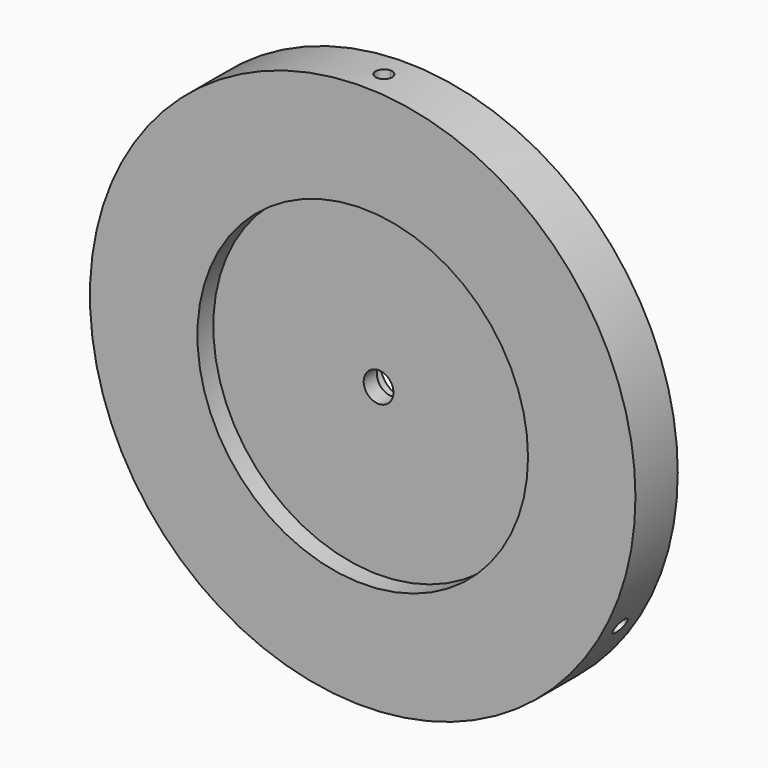
from build123d import *

# Parameters (mm, degrees)
F0_R            = 82.5
F1_DEPTH        = 16
F2_R            = 50
F3_DEPTH        = 6
F6_DEPTH        = 28
F6_COPIES_COUNT = 3
F7_R            = 4.5
F8_DEPTH        = 25
F9_R            = 7.5
F9_R_2          = 4.5
F10_DEPTH       = 5


# Not quite as in the source:
# - a pattern or mirror of a feature is missing from the dataset's text; its kind, count and spacing are read off the source's solid


with BuildPart() as f1:
    # F0 (on Front) → F1 (new body)
    with BuildSketch(Plane.XZ):
        Circle(F0_R)
    extrude(amount=F1_DEPTH)

    # F2 (on face) → F3 (cut)
    with BuildSketch(Plane.XZ.offset(16)):
        Circle(F2_R)
    extrude(amount=-F3_DEPTH, mode=Mode.SUBTRACT)

    # F5 (on offset) → F6 (cut)
    with BuildSketch(Plane.XY.offset(82.5)):
        with BuildLine():
            ThreePointArc((2.5, -8), (1.767766953, -6.232233047), (0, -5.5))
            Line((0, -5.5), (0, -10.5))
            ThreePointArc((0, -10.5), (1.767766953, -9.767766953), (2.5, -8))
        make_face()
        with BuildLine():
            Line((0, -10.5), (0, -5.5))
            ThreePointArc((0, -5.5), (-2.5, -8), (0, -10.5))
        make_face()
    f6 = extrude(amount=-F6_DEPTH, mode=Mode.SUBTRACT)

    # F6_copies: F6 ×3 about axis
    f6_copies_axis = Axis((0, 0, 0), (0, 1, 0))
    for i in range(1, F6_COPIES_COUNT):
        add(f6.rotate(f6_copies_axis, i * 360 / F6_COPIES_COUNT), mode=Mode.SUBTRACT)

    # F7 (on face) → F8 (cut)
    with BuildSketch(Plane.XZ.offset(10)):
        Circle(F7_R)
    extrude(amount=-F8_DEPTH, mode=Mode.SUBTRACT)

    # F9 (on face) → F10 (cut)
    with BuildSketch(Plane(origin=(0, 0, 0), x_dir=(-1, 0, 0), z_dir=(0, 1, 0))):
        Circle(F9_R)
        Circle(F9_R_2, mode=Mode.SUBTRACT)
    extrude(amount=-F10_DEPTH, mode=Mode.SUBTRACT)


solid = f1.part
